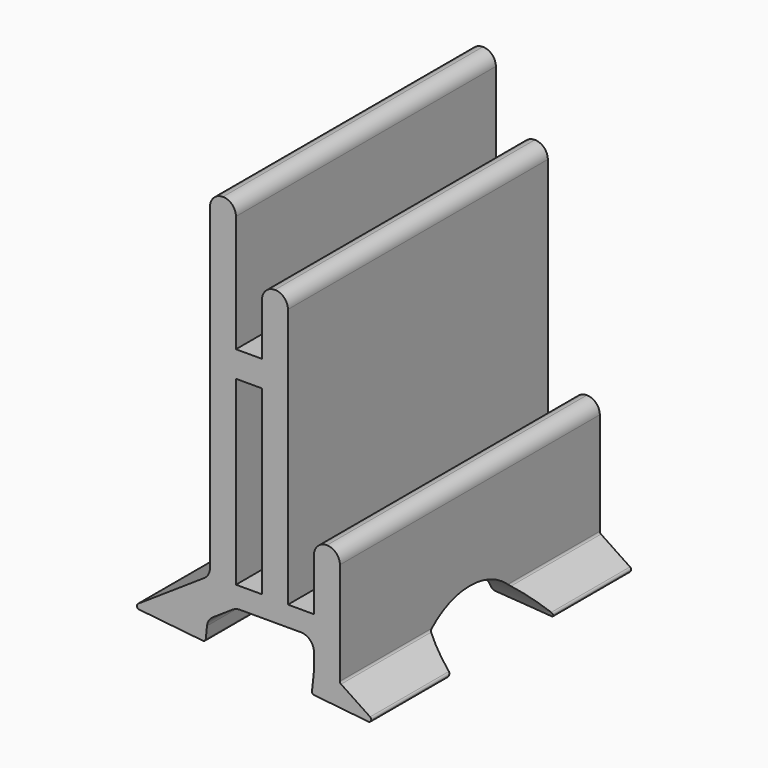
from build123d import *

# Parameters (mm, degrees)
F0_W     = 10
F0_H     = 69.7555384352
F1_DEPTH = 125
F2_R     = 1
F3_R     = 4.99999
F5_R     = 5
F6_R     = 5
F8_R     = 27.5
F9_DEPTH = 128.1414455964


# Not quite as in the source:
# - two fillets or chamfers of one size are made in one step
# - a fillet or chamfer is up to 0.001 mm smaller than in the source, because OpenCascade refuses the exact size


with BuildPart() as f1:
    # F0 (on Front) → F1 (new body)
    with BuildSketch(Plane.XZ):
        Polygon((-50, 150), (-50, 20), (-80, 0), (-51.7332726626, -2.9754449829), (-50.8957943865, 4.9805986405), (-40, 12.2444615648), (-30, 12.2444615648), (-10, 12.2444615648), (-10, 10), (-10, 0.6757781788), (-10.8374782761, -7.2802654446), (15, -10), (0, 0), (0, 45), (-10, 45), (-10, 20), (-20, 20), (-20, 125), (-30, 125), (-30, 100), (-40, 100), (-40, 150), align=None)
        with Locations((-35, 55.1222307824)):
            Rectangle(F0_W, F0_H, mode=Mode.SUBTRACT)
    extrude(amount=F1_DEPTH)

    # F2
    f2_edges = [f1.edges().sort_by_distance(p)[0] for p in [
        (-80, -62.5, 0),
        (-10.837478, -62.5, -7.280265),
        (15, -62.5, -10),
        (-51.733273, -62.5, -2.975445),
        (0, -62.5, 0),
    ]]
    fillet(f2_edges, radius=F2_R)

    # F3 (radius 5 in the source; OpenCascade refuses exactly that, so slightly less here)
    f3_edges = [f1.edges().sort_by_distance(p)[0] for p in [
        (0, -62.5, 45),
        (-10, -62.5, 45),
        (-20, -62.5, 125),
        (-30, -62.5, 125),
        (-40, -62.5, 150),
        (-50, -62.5, 150),
    ]]
    fillet(f3_edges, radius=F3_R)

    # F5
    f5_edges = [f1.edges().sort_by_distance(p)[0] for p in [
        (-50.895794, -62.5, 4.980599),
        (-40, -62.5, 12.244462),
        (-10, -62.5, 12.244462),
    ]]
    fillet(f5_edges, radius=F5_R)

    # F6
    f6_edges = [f1.edges().sort_by_distance(p)[0] for p in [
        (-50, -62.5, 20),
    ]]
    fillet(f6_edges, radius=F6_R)

    # F8 (on offset) → F9 (cut, through all)
    with BuildSketch(Plane.YZ.offset(50)):
        with Locations((-62.5, -20)):
            Circle(F8_R)
    extrude(amount=-F9_DEPTH, mode=Mode.SUBTRACT)


solid = f1.part
